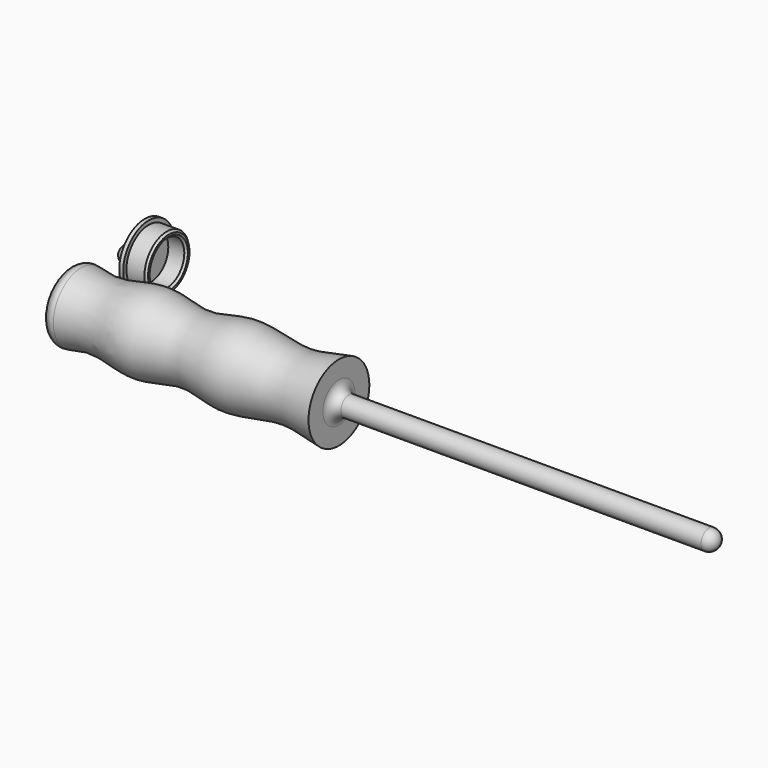
from build123d import *

# Parameters (mm, degrees)
F2_R      = 5
F3_R      = 10
F4_DEPTH  = 128
F9_R      = 10.95
F10_DEPTH = 9
F11_SIZE  = 1


# Not quite as in the source:
# - a feature of the source that left no trace in its solid (it failed there, or was rolled back) is left out


with BuildPart() as f1:
    # F0 (on Top) → F1 (revolve)
    with BuildSketch(Plane.XY):
        with BuildLine():
            Line((0, 19), (0, 0))
            Line((0, 0), (135, 0))
            Line((135, 0), (325, 0))
            Line((325, 0), (325, 5))
            Line((325, 5), (135, 5))
            Line((135, 5), (135, 19))
            add(Edge.make_bspline(
                [(0, 19), (6.2298148154, 17.3381037384), (18.9116523982, 13.5198586362), (41.4617916208, 21.987289281), (63.8339880536, 12.8409507176), (84.8789443524, 21.983405638), (111.8259427397, 13.4206624804), (126.1338785408, 17.3073923453), (135, 19)],
                knots=[0, 0, 0, 0, 0.1530474504, 0.3200912758, 0.4861069731, 0.6487473436, 0.8283759765, 1, 1, 1, 1], degree=3))
        make_face()
    revolve(axis=Axis((67.5, 0, 0), (1, 0, 0)))

    # F2
    f2_edges = [f1.edges().sort_by_distance(p)[0] for p in [
        (325, -5, 0),
        (135, -5, 0),
        (230, 5, 0),
        (0, -19, 0),
    ]]
    fillet(f2_edges, radius=F2_R)

    # F3 (on face) → F4 (cut)
    with BuildSketch(Plane(origin=(0, 0, 0), x_dir=(0, -1, 0), z_dir=(-1, 0, 0))):
        Circle(F3_R)
    extrude(amount=-F4_DEPTH, mode=Mode.SUBTRACT)


with BuildPart() as f6:
    # F5 (on Top) → F6 (revolve)
    with BuildSketch(Plane.XY):
        Polygon((-2, 49.9599839872), (0, 49.9599839872), (10, 49.9599839872), (10, 63.9099839872), (0, 63.9099839872), (0, 65.9099839872), (-2, 65.9099839872), (-2, 58.2169018066), align=None)
    revolve(axis=Axis((-1, 49.9599839872, 0), (1, 0, 0)))

    # F8: sweep along a path in F5
    with BuildLine(Plane.XY) as f8_path:
        ThreePointArc((-2, 41.7030661678), (-10.2569178194, 49.9599839872), (-2, 58.2169018066))
    # F7 (on face) → F8 (sweep)
    with BuildSketch(Plane(origin=(-2, 0, 0), x_dir=(0, -1, 0), z_dir=(-1, 0, 0))):
        with BuildLine():
            ThreePointArc((-43.8375558203, 0), (-41.6849839872, -2.1525718331), (-39.5324121541, 0))
            ThreePointArc((-39.5324121541, 0), (-41.6849839872, 2.1525718331), (-43.8375558203, 0))
        make_face()
    sweep(path=f8_path.line)

    # F9 (on face) → F10 (cut)
    with BuildSketch(Plane.YZ.offset(10)):
        with Locations((49.9599839872, 0)):
            Circle(F9_R)
    extrude(amount=-F10_DEPTH, mode=Mode.SUBTRACT)

    # F11
    f11_edges = [f6.edges().sort_by_distance(p)[0] for p in [
        (10, 36.009984, 0),
        (10, 39.009984, 0),
    ]]
    chamfer(f11_edges, length=F11_SIZE)


solid = Compound([f1.part, f6.part])
